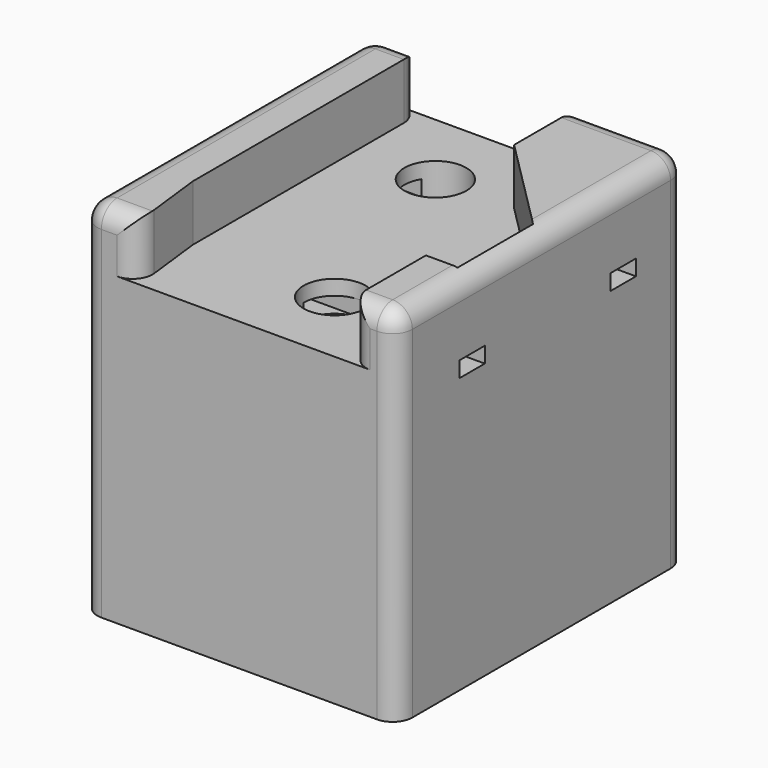
from build123d import *

# Parameters (mm, degrees)
F1_DEPTH     = 58.3
F3_DEPTH     = 9.017
F4_W         = 5.08
F4_H         = 2.54
F5_DEPTH     = 50.801
F6_T1_DEPTH  = 17.9471724254
F6_T3_DEPTH  = 16.9545
F6_T5_DEPTH  = 52.07
F6_T7_DEPTH  = 22.3848784961
F6_T9_DEPTH  = 12.2248784961
F6_T11_DEPTH = 14.0401215039
F6_T13_DEPTH = 12.5401215039
F6_T16_ANGLE = 90
F6_T18_ANGLE = 90
F6_T20_ANGLE = 90
F6_T22_ANGLE = 90
F7_R         = 5
F8_DEPTH     = 25.4
F9_R         = 2.25
F10_DEPTH    = 49.284


# Not quite as in the source:
# - a fillet or chamfer that OpenCascade refuses, or shapes differently, is made with other operations: its cross-section is extruded or revolved along the edge and cut away or added


with BuildPart() as f1:
    # F0 (on Top) → F1 (new body)
    with BuildSketch(Plane.XY):
        with BuildLine():
            Line((47.625, 58.42), (3.175, 58.42))
            ThreePointArc((3.175, 58.42), (0.9299359697, 57.4900640303), (0, 55.245))
            Line((0, 55.245), (0, 3.175))
            ThreePointArc((0, 3.175), (0.9299359697, 0.9299359697), (3.175, 0))
            Line((3.175, 0), (47.625, 0))
            ThreePointArc((47.625, 0), (49.8700640303, 0.9299359697), (50.8, 3.175))
            Line((50.8, 3.175), (50.8, 55.245))
            ThreePointArc((50.8, 55.245), (49.8700640303, 57.4900640303), (47.625, 58.42))
        make_face()
    extrude(amount=F1_DEPTH)

    # F2 (on face) → F3 (cut)
    with BuildSketch(Plane.XY.offset(58.3)):
        Polygon((33.1776215039, 45.72), (33.1776215039, 58.42), (7.7776215039, 58.42), (7.7776215039, 12.7), (9.2776215039, 0), (43.3376215039, 0), (43.3376215039, 15.24), (48.4176215039, 15.24), (48.4176215039, 30.48), align=None)
    extrude(amount=-F3_DEPTH, mode=Mode.SUBTRACT)

    # F4 (on face) → F5 (cut, through all)
    with BuildSketch(Plane.YZ.offset(50.8)):
        with Locations((15.24, 45.6)):
            Rectangle(F4_W, F4_H)
        with Locations((45.72, 45.6)):
            Rectangle(F4_W, F4_H)
    extrude(amount=-F5_DEPTH, mode=Mode.SUBTRACT)

    # F6: fillet of radius 3.175 on 6 edges, made by hand

    # F6_s2 → F6_t1 (cut)
    with BuildSketch(Plane.XY.offset(49.283)):
        with BuildLine():
            ThreePointArc((5.7055525338, 0), (8.0786339971, 1.0657087996), (8.8586359029, 3.5474114216))
            Line((8.8586359029, 3.5474114216), (9.2776215039, 0))
            Line((9.2776215039, 0), (5.7055525338, 0))
        make_face()
    extrude(amount=F6_T1_DEPTH, mode=Mode.SUBTRACT)

    # F6_s4 → F6_t3 (cut)
    with BuildSketch(Plane.XY.offset(49.283)):
        with BuildLine():
            ThreePointArc((46.5126215039, 0), (44.2675574737, 0.9299359697), (43.3376215039, 3.175))
            Line((43.3376215039, 3.175), (43.3376215039, 0))
            Line((43.3376215039, 0), (46.5126215039, 0))
        make_face()
        with BuildLine():
            ThreePointArc((4.6026215039, 58.42), (6.8476855342, 57.4900640303), (7.7776215039, 55.245))
            Line((7.7776215039, 55.245), (7.7776215039, 58.42))
            Line((7.7776215039, 58.42), (4.6026215039, 58.42))
        make_face()
        with BuildLine():
            ThreePointArc((36.3526215039, 58.42), (34.1075574737, 57.4900640303), (33.1776215039, 55.245))
            Line((33.1776215039, 55.245), (33.1776215039, 58.42))
            Line((33.1776215039, 58.42), (36.3526215039, 58.42))
        make_face()
    extrude(amount=F6_T3_DEPTH, mode=Mode.SUBTRACT)

    # F6_s6 → F6_t5 (cut)
    with BuildSketch(Plane.XZ.offset(-55.245)):
        with BuildLine():
            ThreePointArc((0, 55.125), (0.9299359697, 57.3700640303), (3.175, 58.3))
            Line((3.175, 58.3), (0, 58.3))
            Line((0, 58.3), (0, 55.125))
        make_face()
        with BuildLine():
            ThreePointArc((50.8, 55.125), (49.8700640303, 57.3700640303), (47.625, 58.3))
            Line((47.625, 58.3), (50.8, 58.3))
            Line((50.8, 58.3), (50.8, 55.125))
        make_face()
    extrude(amount=F6_T5_DEPTH, mode=Mode.SUBTRACT)

    # F6_s8 → F6_t7 (cut)
    with BuildSketch(Plane.YZ.offset(25.2401215039)):
        with BuildLine():
            ThreePointArc((55.245, 58.3), (57.4900640303, 57.3700640303), (58.42, 55.125))
            Line((58.42, 55.125), (58.42, 58.3))
            Line((58.42, 58.3), (55.245, 58.3))
        make_face()
    extrude(amount=F6_T7_DEPTH, mode=Mode.SUBTRACT)

    # F6_s10 → F6_t9 (cut)
    with BuildSketch(Plane.YZ.offset(35.4001215039)):
        with BuildLine():
            ThreePointArc((3.175, 58.3), (0.9299359697, 57.3700640303), (0, 55.125))
            Line((0, 55.125), (0, 58.3))
            Line((0, 58.3), (3.175, 58.3))
        make_face()
    extrude(amount=F6_T9_DEPTH, mode=Mode.SUBTRACT)

    # F6_s12 → F6_t11 (cut)
    with BuildSketch(Plane.YZ.offset(3.175)):
        with BuildLine():
            ThreePointArc((0, 55.125), (0.9299359697, 57.3700640303), (3.175, 58.3))
            Line((3.175, 58.3), (0, 58.3))
            Line((0, 58.3), (0, 55.125))
        make_face()
    extrude(amount=F6_T11_DEPTH, mode=Mode.SUBTRACT)

    # F6_s14 → F6_t13 (cut)
    with BuildSketch(Plane.YZ.offset(3.175)):
        with BuildLine():
            ThreePointArc((58.42, 55.125), (57.4900640303, 57.3700640303), (55.245, 58.3))
            Line((55.245, 58.3), (58.42, 58.3))
            Line((58.42, 58.3), (58.42, 55.125))
        make_face()
    extrude(amount=F6_T13_DEPTH, mode=Mode.SUBTRACT)

    # F6_s15 → F6_t16 (revolve, cut)
    with BuildSketch(Plane.YZ.offset(47.625)):
        with BuildLine():
            ThreePointArc((0, 55.125), (0.9299359697, 57.3700640303), (3.175, 58.3))
            Line((3.175, 58.3), (0, 58.3))
            Line((0, 58.3), (0, 55.125))
        make_face()
    revolve(axis=Axis((47.625, 3.175, 58.3), (0, 0, 1)), revolution_arc=F6_T16_ANGLE, mode=Mode.SUBTRACT)

    # F6_s17 → F6_t18 (revolve, cut)
    with BuildSketch(Plane.XZ.offset(-55.245)):
        with BuildLine():
            ThreePointArc((47.625, 58.3), (49.8700640303, 57.3700640303), (50.8, 55.125))
            Line((50.8, 55.125), (50.8, 58.3))
            Line((50.8, 58.3), (47.625, 58.3))
        make_face()
    revolve(axis=Axis((47.625, 55.245, 58.3), (0, 0, 1)), revolution_arc=F6_T18_ANGLE, mode=Mode.SUBTRACT)

    # F6_s19 → F6_t20 (revolve, cut)
    with BuildSketch(Plane.YZ.offset(3.175)):
        with BuildLine():
            ThreePointArc((58.42, 55.125), (57.4900640303, 57.3700640303), (55.245, 58.3))
            Line((55.245, 58.3), (58.42, 58.3))
            Line((58.42, 58.3), (58.42, 55.125))
        make_face()
    revolve(axis=Axis((3.175, 55.245, 58.3), (0, 0, 1)), revolution_arc=F6_T20_ANGLE, mode=Mode.SUBTRACT)

    # F6_s21 → F6_t22 (revolve, cut)
    with BuildSketch(Plane.XZ.offset(-3.175)):
        with BuildLine():
            ThreePointArc((0, 55.125), (0.9299359697, 57.3700640303), (3.175, 58.3))
            Line((3.175, 58.3), (0, 58.3))
            Line((0, 58.3), (0, 55.125))
        make_face()
    revolve(axis=Axis((3.175, 3.175, 58.3), (0, 0, 1)), revolution_arc=F6_T22_ANGLE, mode=Mode.SUBTRACT)

    # F7 (on face) → F8 (cut)
    with BuildSketch(Plane.XY.offset(49.283)):
        with Locations((20.4776215039, 45.72)):
            Circle(F7_R)
        with Locations((30.6376215039, 12.7)):
            Circle(F7_R)
    extrude(amount=-F8_DEPTH, mode=Mode.SUBTRACT)

    # F9 (on face) → F10 (cut, through all)
    with BuildSketch(Plane.XY.offset(49.283)):
        with Locations((20.4776215039, 45.72)):
            Circle(F9_R)
        with Locations((30.6376215039, 12.7)):
            Circle(F9_R)
    extrude(amount=-F10_DEPTH, mode=Mode.SUBTRACT)


solid = f1.part
